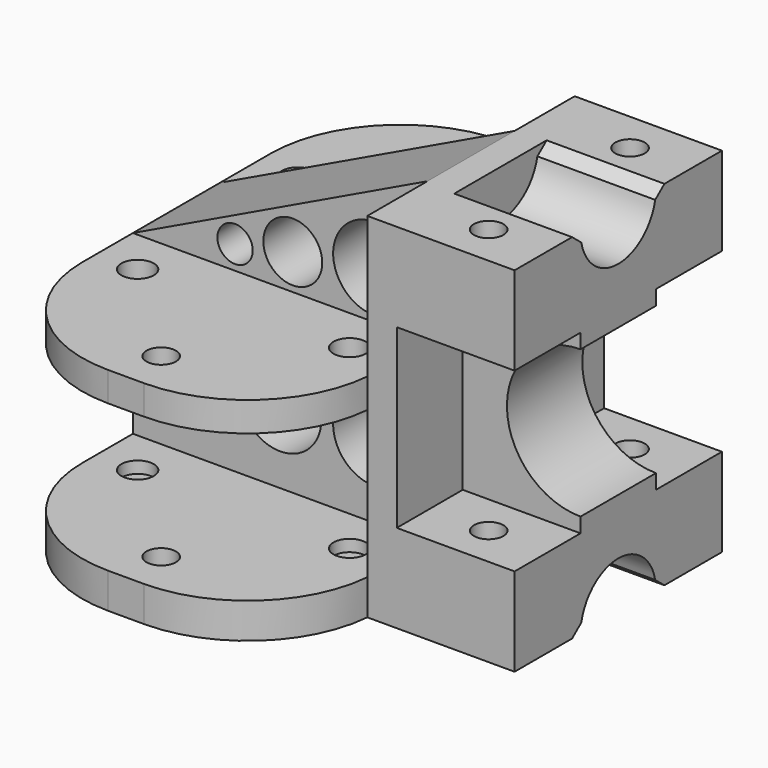
from build123d import *

# Parameters (mm, degrees)
F0_W         = 25
F0_H         = 44
F1_DEPTH     = 60
F0_W_2       = 50
F0_H_2       = 20
F0_R         = 2.5
F2_DEPTH     = 6
F3_R         = 8
F4_DEPTH     = 20
F5_R         = 2.5
F6_DEPTH     = 60
F7_W         = 14
F7_H         = 30
F8_DEPTH     = 20
F9_START     = 25
F2_FACE_R    = 2.5
F9_DEPTH     = 5
F10_T1_DEPTH = 114.544511501
F10_T3_DEPTH = 115.544511501
F10_T5_DEPTH = 116
F10_T7_DEPTH = 115
F11_R        = 2.75
F12_DEPTH    = 32
F13_W        = 50
F13_H        = 18.5
F14_DEPTH    = 54
F16_DEPTH    = 18.5
F17_R        = 12.5
F18_DEPTH    = 16.8
F19_R        = 7
F20_DEPTH    = 18.5
F21_R        = 7
F21_R_2      = 3
F21_R_3      = 5
F22_DEPTH    = 18.5
F23_T1_DEPTH = 24.6515369414


# Not quite as in the source:
# - a fillet or chamfer that OpenCascade refuses, or shapes differently, is made with other operations: its cross-section is extruded or revolved along the edge and cut away or added


with BuildPart() as f1:
    # F0 (on Top) → F1 (new body)
    with BuildSketch(Plane.XY):
        with Locations((37.5, 0)):
            Rectangle(F0_W, F0_H)
    extrude(amount=F1_DEPTH)

    # F0 (on Top) → F2 (join)
    with BuildSketch(Plane.XY):
        with Locations((0, 32)):
            Rectangle(F0_W_2, F0_H_2)
        with Locations((0, 34.5)):
            Circle(F0_R, mode=Mode.SUBTRACT)
        Rectangle(F0_W_2, F0_H)
        with Locations((0, -32)):
            Rectangle(F0_W_2, F0_H_2)
        with Locations((0, -34.5)):
            Circle(F0_R, mode=Mode.SUBTRACT)
    extrude(amount=F2_DEPTH)

    # F3 (on face) → F4 (cut)
    with BuildSketch(Plane.YZ.offset(50)):
        Circle(F3_R)
        with Locations((0, 60)):
            Circle(F3_R)
    extrude(amount=-F4_DEPTH, mode=Mode.SUBTRACT)

    # F5 (on face) → F6 (cut)
    with BuildSketch(Plane.XY.offset(60)):
        with Locations((40, 15)):
            Circle(F5_R)
        with Locations((40, -15)):
            Circle(F5_R)
    extrude(amount=-F6_DEPTH, mode=Mode.SUBTRACT)

    # F7 (on face) → F8 (cut)
    with BuildSketch(Plane.YZ.offset(50)):
        with Locations((-15, 30)):
            Rectangle(F7_W, F7_H)
        with Locations((15, 30)):
            Rectangle(F7_W, F7_H)
    extrude(amount=-F8_DEPTH, mode=Mode.SUBTRACT)

    # F2_face (on face) → F9 (join)
    with BuildSketch(Plane.XY.offset(6).offset(F9_START)):
        Polygon((-25, 42), (-25, -42), (25, -42), (25, -22), (25, 22), (25, 42), align=None)
        with Locations((0, 34.5)):
            Circle(F2_FACE_R, mode=Mode.SUBTRACT)
        with Locations((0, -34.5)):
            Circle(F2_FACE_R, mode=Mode.SUBTRACT)
    extrude(amount=F9_DEPTH)

    # F10: fillet of radius 22 on 8 edges, made by hand

    # F10_s2 → F10_t1 (cut)
    with BuildSketch(Plane.XY.offset(-23.7722557505)):
        with BuildLine():
            ThreePointArc((25, -22), (17.923494674, -36.2480768093), (3.0910976998, -42))
            Line((3.0910976998, -42), (25, -42))
            Line((25, -42), (25, -22))
        make_face()
        with BuildLine():
            ThreePointArc((25, 22), (17.923494674, 36.2480768093), (3.0910976998, 42))
            Line((3.0910976998, 42), (25, 42))
            Line((25, 42), (25, 22))
        make_face()
    extrude(amount=F10_T1_DEPTH, mode=Mode.SUBTRACT)

    # F10_s4 → F10_t3 (cut)
    with BuildSketch(Plane.XY.offset(-54.7722557505)):
        with BuildLine():
            ThreePointArc((3.0910976998, -42), (17.923494674, -36.2480768093), (25, -22))
            Line((25, -22), (25, -42))
            Line((25, -42), (3.0910976998, -42))
        make_face()
        with BuildLine():
            ThreePointArc((25, 22), (17.923494674, 36.2480768093), (3.0910976998, 42))
            Line((3.0910976998, 42), (25, 42))
            Line((25, 42), (25, 22))
        make_face()
    extrude(amount=F10_T3_DEPTH, mode=Mode.SUBTRACT)

    # F10_s6 → F10_t5 (cut)
    with BuildSketch(Plane.XY.offset(-55)):
        with BuildLine():
            ThreePointArc((-25, -20), (-18.5563491861, -35.5563491861), (-3, -42))
            Line((-3, -42), (-25, -42))
            Line((-25, -42), (-25, -20))
        make_face()
        with BuildLine():
            ThreePointArc((-3, 42), (-18.5563491861, 35.5563491861), (-25, 20))
            Line((-25, 20), (-25, 42))
            Line((-25, 42), (-3, 42))
        make_face()
    extrude(amount=F10_T5_DEPTH, mode=Mode.SUBTRACT)

    # F10_s8 → F10_t7 (cut)
    with BuildSketch(Plane.XY.offset(-24)):
        with BuildLine():
            ThreePointArc((-25, -20), (-18.5563491861, -35.5563491861), (-3, -42))
            Line((-3, -42), (-25, -42))
            Line((-25, -42), (-25, -20))
        make_face()
        with BuildLine():
            ThreePointArc((-3, 42), (-18.5563491861, 35.5563491861), (-25, 20))
            Line((-25, 20), (-25, 42))
            Line((-25, 42), (-3, 42))
        make_face()
    extrude(amount=F10_T7_DEPTH, mode=Mode.SUBTRACT)

    # F11 (on face) → F12 (cut)
    with BuildSketch(Plane.XY.offset(36)):
        with Locations((18, 17)):
            Circle(F11_R)
        with Locations((-18, 17)):
            Circle(F11_R)
        with Locations((-18, -17)):
            Circle(F11_R)
        with Locations((18, -17)):
            Circle(F11_R)
    extrude(amount=-F12_DEPTH, mode=Mode.SUBTRACT)

    # F13 (on face) → F14 (join)
    with BuildSketch(Plane.XY.offset(6)):
        Rectangle(F13_W, F13_H)
    extrude(amount=F14_DEPTH)

    # F15 (on face) → F16 (cut)
    with BuildSketch(Plane.XZ.offset(9.25)):
        Polygon((-25, 36), (25, 60), (-25, 60), align=None)
    extrude(amount=-F16_DEPTH, mode=Mode.SUBTRACT)

    # F17 (on face) → F18 (cut)
    with BuildSketch(Plane.XZ.offset(8)):
        with Locations((50, 30)):
            Circle(F17_R)
    extrude(amount=-F18_DEPTH, mode=Mode.SUBTRACT)

    # F19 (on face) → F20 (cut)
    with BuildSketch(Plane.XZ.offset(9.25)):
        with Locations((0, 18.5)):
            Circle(F19_R)
        with Locations((16, 18.5)):
            Circle(F19_R)
        with Locations((-16, 18.5)):
            Circle(F19_R)
    extrude(amount=-F20_DEPTH, mode=Mode.SUBTRACT)

    # F21 (on face) → F22 (cut)
    with BuildSketch(Plane.XZ.offset(9.25)):
        with Locations((16, 44)):
            Circle(F21_R)
        with Locations((-7.6543654317, 40)):
            Circle(F21_R_2)
        with Locations((2.1435935394, 42)):
            Circle(F21_R_3)
    extrude(amount=-F22_DEPTH, mode=Mode.SUBTRACT)

    # F23: chamfer of 2 on 4 edges, made by hand

    # F23_s2 → F23_t1 (cut)
    with BuildSketch(Plane.YZ.offset(30)):
        with BuildLine():
            Line((9.7979589711, 60), (7.8383671769, 58.4))
            ThreePointArc((7.8383671769, 58.4), (7.9565711479, 59.1675484588), (8, 60))
            Line((8, 60), (9.7979589711, 60))
        make_face()
        with BuildLine():
            Line((-9.7979589711, 60), (-7.8383671769, 58.4))
            ThreePointArc((-7.8383671769, 58.4), (-7.9565711479, 59.1675484588), (-8, 60))
            Line((-8, 60), (-9.7979589711, 60))
        make_face()
        with BuildLine():
            Line((9.7979589711, 0), (7.8383671769, 1.6))
            ThreePointArc((7.8383671769, 1.6), (7.9565711479, 0.8324515412), (8, 0))
            Line((8, 0), (9.7979589711, 0))
        make_face()
        with BuildLine():
            Line((-9.7979589711, 0), (-7.8383671769, 1.6))
            ThreePointArc((-7.8383671769, 1.6), (-7.9565711479, 0.8324515412), (-8, 0))
            Line((-8, 0), (-9.7979589711, 0))
        make_face()
    extrude(amount=F23_T1_DEPTH, mode=Mode.SUBTRACT)


solid = f1.part
